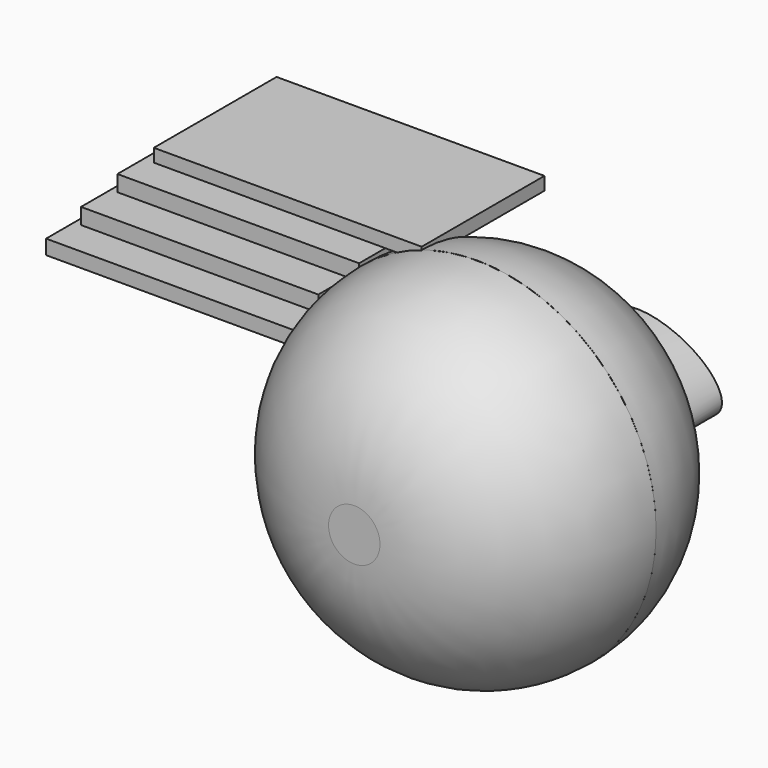
from build123d import *

# Parameters (mm, degrees)
F0_R     = 29.6579287445
F1_DEPTH = 50.8
F2_R     = 25.39999
F3_R     = 7.026121943
F3_W     = 44.3428866565
F3_H     = 2.1689496934
F3_W_2   = 40.0050021708
F3_H_2   = 2.6509352028
F3_W_3   = 39.2820164561
F3_H_3   = 2.6509370655
F5_DEPTH = 25.4
F3_W_4   = 42.4149371684
F3_H_4   = 2.4099387228


# Not quite as in the source:
# - a fillet or chamfer is up to 0.001 mm smaller than in the source, because OpenCascade refuses the exact size
# - the program builds the solid bodies; features that only make, move or delete a surface that nothing else refers to are left out


with BuildPart() as f1:
    # F0 (on Front) → F1 (new body)
    with BuildSketch(Plane.XZ):
        with Locations((-22.4124398082, 11.8087045848)):
            Circle(F0_R)
    extrude(amount=F1_DEPTH)

    # F2 (radius 25.4 in the source; OpenCascade refuses exactly that, so slightly less here)
    f2_edges = [f1.edges().sort_by_distance(p)[0] for p in [
        (-52.070369, -50.8, 11.808705),
        (-52.070369, 0, 11.808705),
    ]]
    fillet(f2_edges, radius=F2_R)

    # F3 (on Front) → F5 (join)
    with BuildSketch(Plane.XZ):
        with BuildLine():
            add(Edge.make_bspline(
                [(-33.2571677864, 27.9553029686), (-37.1422937885, 31.7064598227), (-45.3214823641, 19.3476406869), (-53.5006709397, 6.9888215512), (-41.436356362, 15.5964838329), (-29.3720417843, 24.2041461146), (-33.2571677864, 27.9553029686)],
                knots=[0, 0, 0, 2.0943951024, 2.0943951024, 4.1887902048, 4.1887902048, 6.2831853072, 6.2831853072, 6.2831853072], degree=2, weights=[1, 0.5, 1, 0.5, 1, 0.5, 1]))
        make_face()
        with BuildLine():
            add(Edge.make_bspline(
                [(-2.4099403527, 15.9056037664), (1.0870038831, 23.7223034997), (-14.398125451, 25.9592996115), (-29.8832547851, 28.1962957233), (-17.8950696867, 18.1425998783), (-5.9068845884, 8.0889040332), (-2.4099403527, 15.9056037664)],
                knots=[0, 0, 0, 2.0943951024, 2.0943951024, 4.1887902048, 4.1887902048, 6.2831853072, 6.2831853072, 6.2831853072], degree=2, weights=[1, 0.5, 1, 0.5, 1, 0.5, 1]))
        make_face()
        with Locations((-25.5453623831, -7.2298194282)):
            Circle(F3_R)
        with Locations((-53.7416581064, 39.4025165588)):
            Rectangle(F3_W, F3_H)
        with Locations((-61.9354527444, 33.377667889)):
            Rectangle(F3_W_2, F3_H_2)
        with Locations((-68.3217905462, 26.6298344359)):
            Rectangle(F3_W_3, F3_H_3)
    extrude(amount=F5_DEPTH)


with BuildPart() as f5:
    # F3 (on Front) → F5, piece 2 (new body)
    with BuildSketch(Plane.XZ):
        with Locations((-72.5391861051, 20.2434938401)):
            Rectangle(F3_W_4, F3_H_4)
    extrude(amount=F5_DEPTH)


solid = Compound([f1.part, f5.part])
